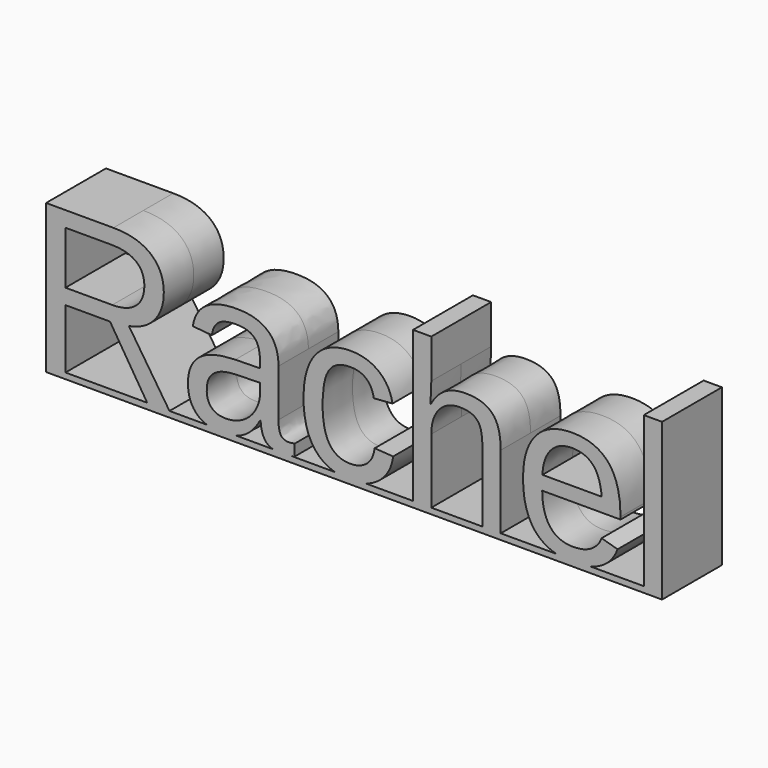
from build123d import *

# Parameters (mm, degrees)
F0_TEXT_SIZE = 35.2777777778
F1_DEPTH     = 6.35
F2_W         = 104.5545138889
F2_H         = 12.7
F3_DEPTH     = 1


# Not quite as in the source:
# - Text() gives the source's letters only with a copy of the font that has no kerning and outlines rounded to 1/6400 em; it was checked with that copy


with BuildPart() as f1:
    # F0 (on Front) → F1 (new body, symmetric)
    with BuildSketch(Plane.XZ):
        with Locations((-54.9478949653, 0)):
            Text('Rachel', F0_TEXT_SIZE, font='Arimo', text_align=(TextAlign.LEFT, TextAlign.BOTTOM))
    extrude(amount=F1_DEPTH, both=True)

    # F2 (on Top) → F3 (join)
    with BuildSketch(Plane.XY):
        with Locations((0.2232421875, 0)):
            Rectangle(F2_W, F2_H)
    extrude(amount=-F3_DEPTH)


solid = f1.part
